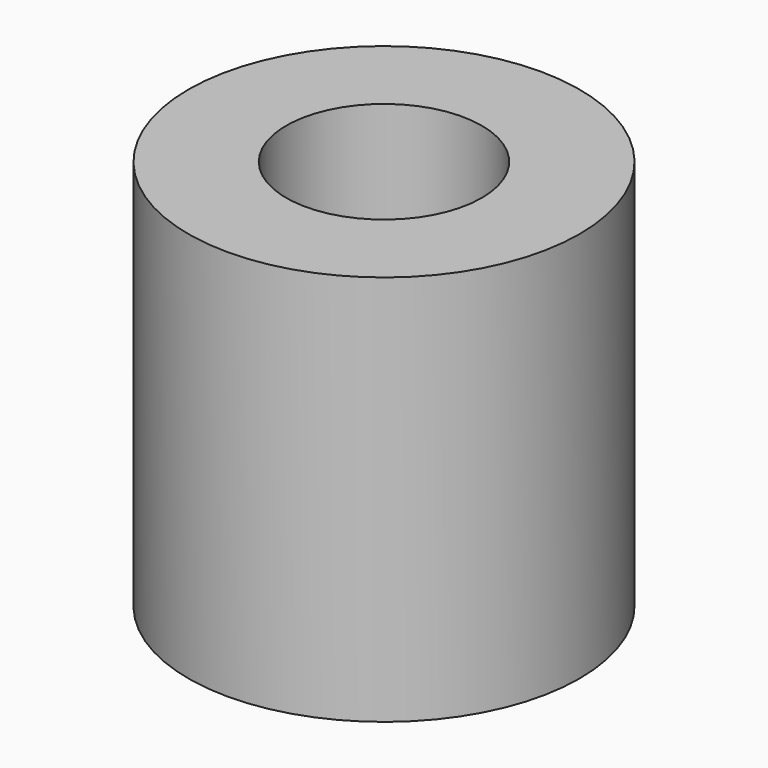
from build123d import *

# Parameters (mm, degrees)
F0_R     = 4.7625
F0_R_2   = 2.38125
F1_DEPTH = 9.525


# Not quite as in the source:
# - a length typed as a fraction of an inch, garbled in the dataset ("3 / 203.2 mm" for 3/8 in), is restored


with BuildPart() as f1:
    # F0 (on Top) → F1 (new body)
    with BuildSketch(Plane.XY):
        Circle(F0_R)
        Circle(F0_R_2, mode=Mode.SUBTRACT)
    extrude(amount=F1_DEPTH)


solid = f1.part
